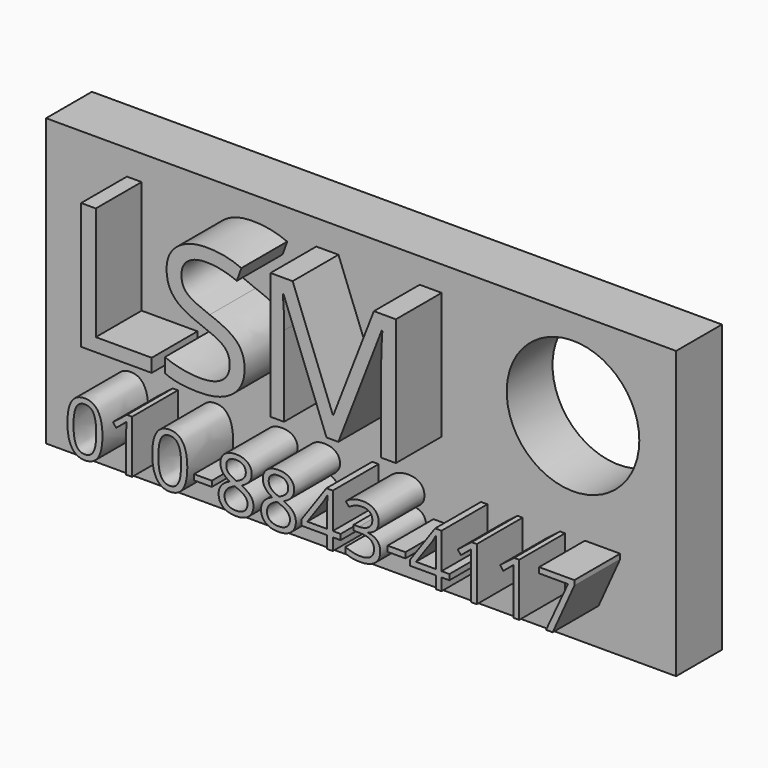
from build123d import *

# Parameters (mm, degrees)
F0_W           = 55
F0_H           = 25
F1_DEPTH       = 5
F2_TEXT_SIZE   = 15.480125776
F2_TEXT_SIZE_2 = 6.478169917
F3_DEPTH       = 5
F4_R           = 5.7879643
F5_DEPTH       = 25


# Not quite as in the source:
# - Text() gives the source's letters only with a copy of the font that has no kerning and outlines rounded to 1/6400 em; it was checked with that copy


with BuildPart() as f1:
    # F0 (on Front) → F1 (new body)
    with BuildSketch(Plane.XZ):
        with Locations((27.5, 12.5)):
            Rectangle(F0_W, F0_H)
    extrude(amount=F1_DEPTH)

    # F2 (on face) → F3 (join)
    with BuildSketch(Plane.XZ.offset(5)):
        with Locations((5.5388350214, 11.7578792733)):
            Text('LSM', F2_TEXT_SIZE, font='Open Sans', text_align=(TextAlign.LEFT, TextAlign.BOTTOM))
        with Locations((5.5388350214, 3.2066939725)):
            Text('010-8843-4117', F2_TEXT_SIZE_2, font='Open Sans', text_align=(TextAlign.LEFT, TextAlign.BOTTOM))
    extrude(amount=F3_DEPTH)

    # F4 (on face) → F5 (cut)
    with BuildSketch(Plane.XZ.offset(5)):
        with Locations((45.9997057915, 17.0749425888)):
            Circle(F4_R)
    extrude(amount=-F5_DEPTH, mode=Mode.SUBTRACT)


solid = f1.part
